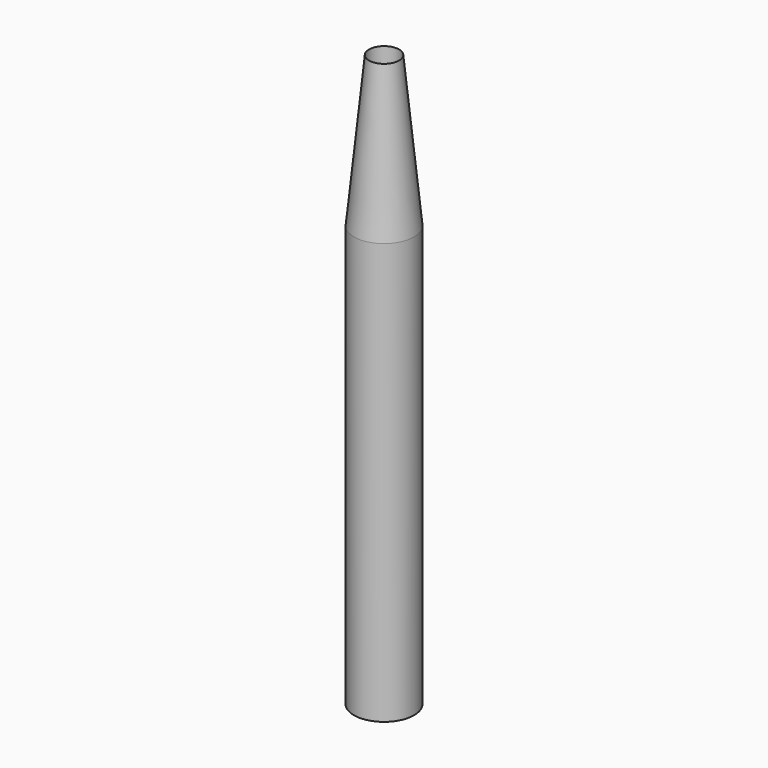
from build123d import *

# Parameters (mm, degrees)
F0_R     = 1
F0_R_2   = 0.5
F1_DEPTH = 19
F2_SIZE2 = 4.99999
F2_SIZE  = 0.49999


# Not quite as in the source:
# - a fillet or chamfer is up to 0.001 mm smaller than in the source, because OpenCascade refuses the exact size


with BuildPart() as f1:
    # F0 (on Top) → F1 (new body)
    with BuildSketch(Plane.XY):
        Circle(F0_R)
        Circle(F0_R_2, mode=Mode.SUBTRACT)
    extrude(amount=F1_DEPTH)

    # F2 (size 0.5 and 5 in the source; OpenCascade refuses exactly that, so slightly less here)
    f2_edges = [f1.edges().sort_by_distance(p)[0] for p in [
        (-1, 0, 19),
    ]]
    f2_side = f1.faces().sort_by_distance((-0.971716, 0, 19))[0]
    chamfer(f2_edges, length=F2_SIZE, length2=F2_SIZE2, reference=f2_side)


solid = f1.part
